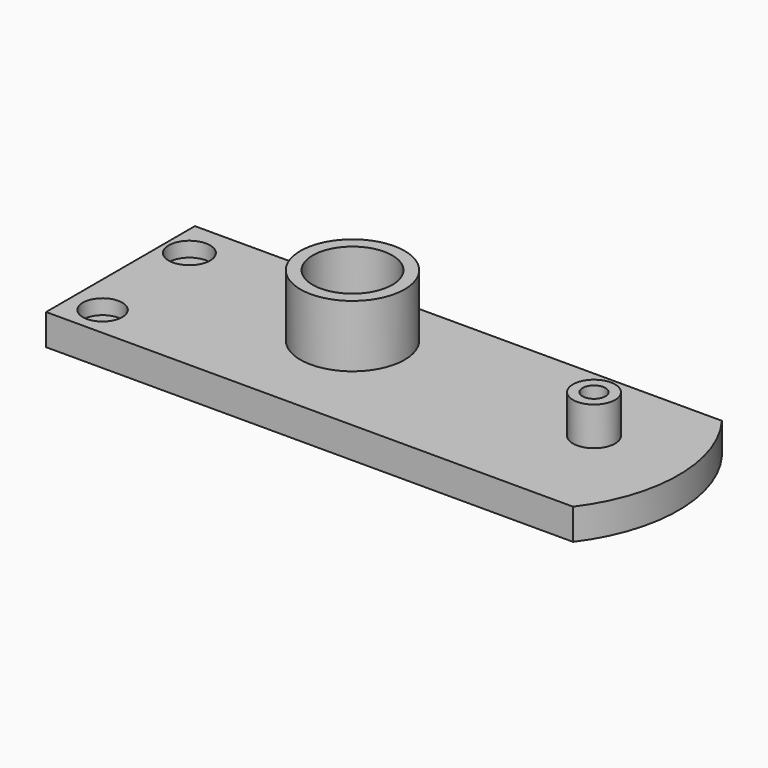
from build123d import *

# Parameters (mm, degrees)
F1_DEPTH  = 12.7
F2_R      = 21.351508313
F5_DEPTH  = 25.4
F3_R      = 8.6303522865
F6_DEPTH  = 15.748
F7_R      = 16.3268483507
F8_DEPTH  = 25.4
F9_R      = 4.6742871789
F10_DEPTH = 25.4
F12_R     = 8.0691836116
F13_DEPTH = 6.096
F14_R     = 8.4816227384
F15_DEPTH = 6.096
F16_R     = 7.7449040589
F16_R_2   = 7.9980791945
F17_DEPTH = 9.906
F20_DEPTH = 76.2
F22_DEPTH = 54.61


with BuildPart() as f1:
    # F0 (on Top) → F1 (new body)
    with BuildSketch(Plane.XY):
        with BuildLine():
            Line((43.0717023765, 44.353062627), (-172.8282976235, 44.353062627))
            Line((-172.8282976235, 44.353062627), (-172.8282976235, -31.846937373))
            Line((-172.8282976235, -31.846937373), (43.0717023765, -31.846937373))
            ThreePointArc((43.0717023765, -31.846937373), (55.7717023765, 6.253062627), (43.0717023765, 44.353062627))
        make_face()
    extrude(amount=F1_DEPTH)

    # F2 (on face) → F5 (join)
    with BuildSketch(Plane.XY.offset(12.7)):
        with Locations((-83.9282976235, 13.9431571588)):
            Circle(F2_R)
    extrude(amount=F5_DEPTH)

    # F3 (on face) → F6 (join)
    with BuildSketch(Plane.XY.offset(12.7)):
        with Locations((17.6193086471, 10.6806947875)):
            Circle(F3_R)
    extrude(amount=F6_DEPTH)

    # F7 (on face) → F8 (cut)
    with BuildSketch(Plane.XY.offset(38.1)):
        with Locations((-83.9282976235, 13.9431571588)):
            Circle(F7_R)
    extrude(amount=-F8_DEPTH, mode=Mode.SUBTRACT)

    # F9 (on face) → F10 (cut)
    with BuildSketch(Plane.XY.offset(28.448)):
        with Locations((17.6193086471, 10.6806947875)):
            Circle(F9_R)
    extrude(amount=-F10_DEPTH, mode=Mode.SUBTRACT)

    # F12 (on face) → F13 (cut)
    with BuildSketch(Plane.XY.offset(12.7)):
        with Locations((-159.6309095621, -19.4137375802)):
            Circle(F12_R)
    extrude(amount=-F13_DEPTH, mode=Mode.SUBTRACT)

    # F14 (on face) → F15 (cut)
    with BuildSketch(Plane.XY.offset(12.7)):
        with Locations((-162.579163909, 28.7375189364)):
            Circle(F14_R)
    extrude(amount=-F15_DEPTH, mode=Mode.SUBTRACT)

    # F16 (on face) → F17 (join)
    with BuildSketch(Plane.XY.offset(12.7)):
        with Locations((-135.2781951427, 29.6167228371)):
            Circle(F16_R)
        with Locations((-135.2781951427, -19.9670530856)):
            Circle(F16_R_2)
    extrude(amount=-F17_DEPTH)

    # F19 (on face) → F20 (cut)
    with BuildSketch(Plane(origin=(-0.7380402899, 10.8379946946, 0), x_dir=(-0.9976893986, -0.0679401489, 0), z_dir=(-0.0679401489, 0.9976893986, 0))):
        Polygon((-10.0049076565, 30.4591804743), (62.7737756253, 41.8267212808), (62.7737756253, 54.864), (-10.0049076565, 54.864), align=None)
    extrude(amount=F20_DEPTH, mode=Mode.SUBTRACT)

    # F21 (on face) → F22 (cut)
    with BuildSketch(Plane(origin=(1.6560066854, 12.5212517744, 0), x_dir=(0.9913673033, -0.1311139582, 0), z_dir=(-0.1311139582, -0.9913673033, 0))):
        Polygon((7.6538164039, 54.864), (-65.4252028626, 54.864), (7.6538164039, 28.5761542618), align=None)
    extrude(amount=F22_DEPTH, mode=Mode.SUBTRACT)


solid = f1.part
